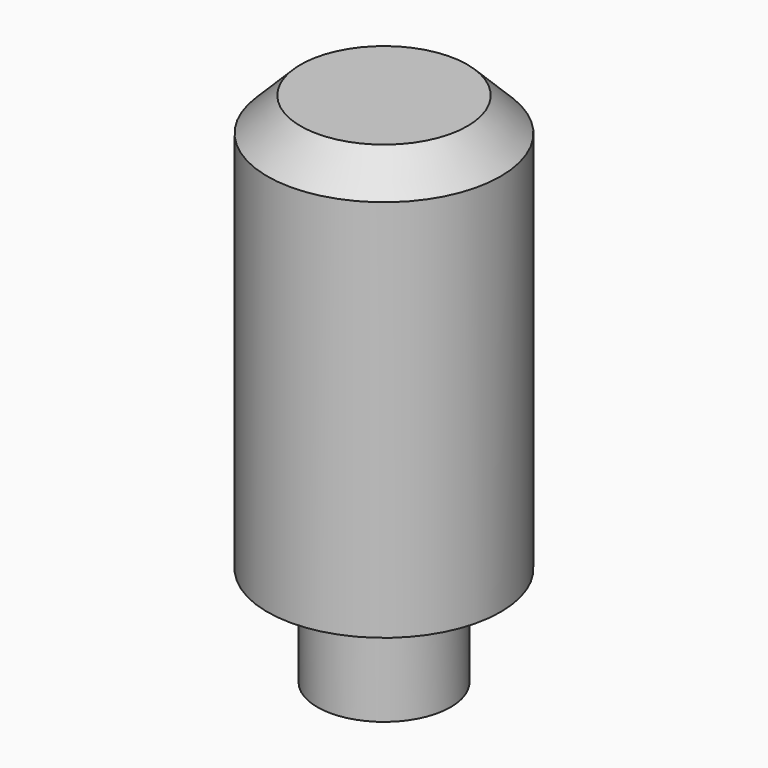
from build123d import *

# Parameters (mm, degrees)
F0_R     = 7
F1_DEPTH = 12.5
F2_SIZE  = 2
F3_R     = 4
F4_DEPTH = 6


with BuildPart() as f1:
    # F0 (on Top) → F1 (new body, symmetric)
    with BuildSketch(Plane.XY):
        Circle(F0_R)
    extrude(amount=F1_DEPTH, both=True)

    # F2
    f2_edges = [f1.edges().sort_by_distance(p)[0] for p in [
        (-7, 0, 12.5),
    ]]
    chamfer(f2_edges, length=F2_SIZE)

    # F3 (on face) → F4 (join)
    with BuildSketch(Plane(origin=(0, 0, -12.5), x_dir=(1, 0, 0), z_dir=(0, 0, -1))):
        Circle(F3_R)
    extrude(amount=F4_DEPTH)


solid = f1.part
